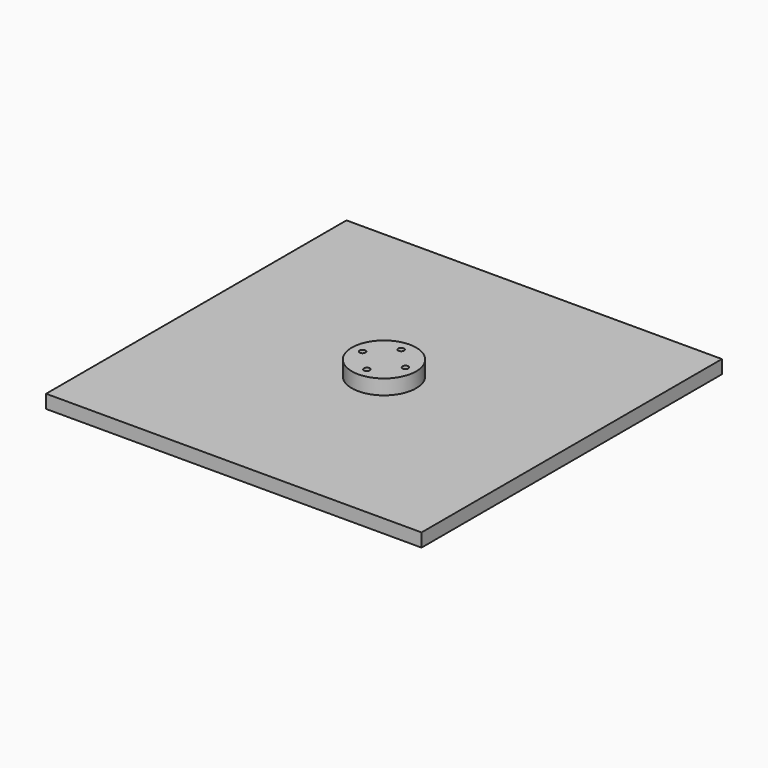
from build123d import *

# Parameters (mm, degrees)
F0_W           = 140
F0_H           = 140
F0_R           = 12
F1_DEPTH       = 5
F2_DEPTH       = 10.56
F3_D           = 2.2
F3_DEPTH       = 12
F3_CBORE_D     = 4
F3_CBORE_DEPTH = 8
F3_TIP         = 0.6609466809


# Not quite as in the source:
# - a feature names something its author has since deleted; it is built from what else it names


with BuildPart() as f1:
    # F0 (on Top) → F1 (new body)
    with BuildSketch(Plane.XY):
        Rectangle(F0_W, F0_H)
        Circle(F0_R, mode=Mode.SUBTRACT)
    extrude(amount=F1_DEPTH)

    # F0 (on Top) → F2 (join)
    with BuildSketch(Plane.XY):
        Circle(F0_R)
    extrude(amount=F2_DEPTH)

    # F3
    with Locations(Plane(origin=(0, 0, 0), x_dir=(1, 0, 0), z_dir=(0, 0, -1))):
        with Locations((8, 0), (0, -8), (-8, 0), (0, 8)):
            CounterBoreHole(F3_D / 2, F3_CBORE_D / 2, F3_CBORE_DEPTH, depth=F3_DEPTH)
            with Locations((0, 0, -(F3_DEPTH + F3_TIP / 2))):  # 118° drill point
                Cone(0, F3_D / 2, F3_TIP, mode=Mode.SUBTRACT)


solid = f1.part
